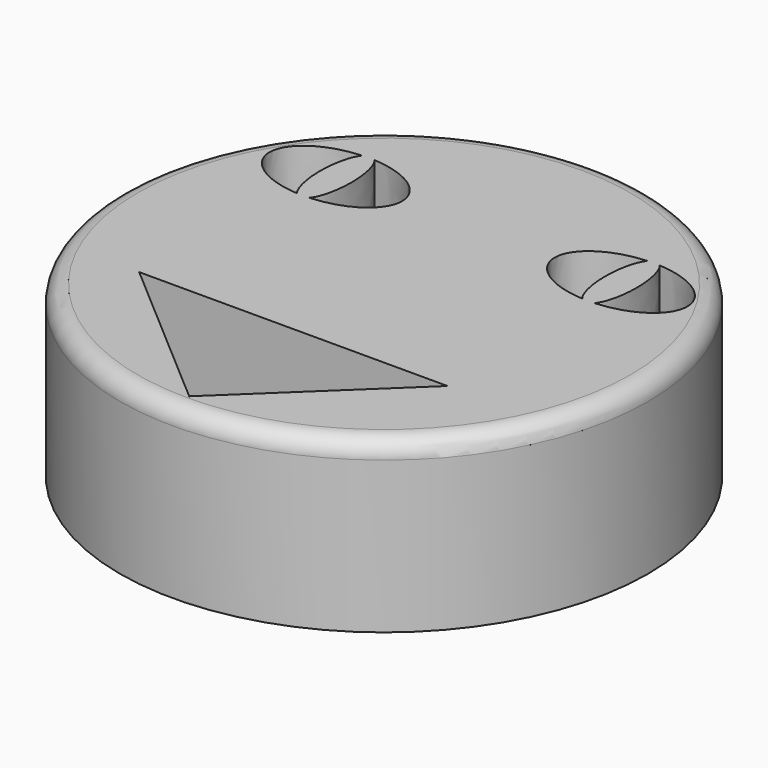
from build123d import *

# Parameters (mm, degrees)
F0_R     = 75.6558411923
F1_DEPTH = 48.514
F2_R     = 5.08


with BuildPart() as f1:
    # F0 (on Top) → F1 (new body)
    with BuildSketch(Plane.XY):
        Circle(F0_R)
        Polygon((0, -69.7530433536), (-46.3102683425, -29.7708865255), (41.9956482947, -29.7708865255), align=None, mode=Mode.SUBTRACT)
        with BuildLine():
            add(Edge.make_bspline(
                [(-21.8607485294, 33.7978675961), (-21.8607485294, 44.4959185344), (-39.0945518587, 45.4823768148)],
                knots=[0, 0, 0, 1.4784559967, 1.4784559967, 1.4784559967], degree=2, weights=[1, 0.73898889, 1]))
            add(Edge.make_bspline(
                [(-39.0945518587, 22.1133583775), (-21.8607485294, 23.0998166579), (-21.8607485294, 33.7978675961)],
                knots=[4.8047293104, 4.8047293104, 4.8047293104, 6.2831853072, 6.2831853072, 6.2831853072], degree=2, weights=[1, 0.73898889, 1]))
            add(Edge.make_bspline(
                [(-40.8450812101, 21.1076120934), (-39.9337015522, 21.1076120934), (-39.0945518587, 22.1133583775)],
                knots=[0, 0, 0, 0.4008066518, 0.4008066518, 0.4008066518], degree=2, weights=[1, 0.9799863696, 1]))
            add(Edge.make_bspline(
                [(-42.5956105616, 22.1133583775), (-41.7564608681, 21.1076120934), (-40.8450812101, 21.1076120934)],
                knots=[5.8823786554, 5.8823786554, 5.8823786554, 6.2831853072, 6.2831853072, 6.2831853072], degree=2, weights=[1, 0.9799863696, 1]))
            add(Edge.make_bspline(
                [(-42.5956105616, 45.4823768148), (-59.8294138908, 44.4959185344), (-59.8294138908, 33.7978675961), (-59.8294138908, 23.0998166579), (-42.5956105616, 22.1133583775)],
                knots=[1.6631366568, 1.6631366568, 1.6631366568, 3.1415926536, 3.1415926536, 4.6200486503, 4.6200486503, 4.6200486503], degree=2, weights=[1, 0.73898889, 1, 0.73898889, 1]))
            add(Edge.make_bspline(
                [(-39.0945518587, 45.4823768148), (-40.8450812101, 47.5804391797), (-42.5956105616, 45.4823768148)],
                knots=[2.7407860018, 2.7407860018, 2.7407860018, 3.5423993054, 3.5423993054, 3.5423993054], degree=2, weights=[1, 0.9207465694, 1]))
        make_face(mode=Mode.SUBTRACT)
        with BuildLine():
            add(Edge.make_bspline(
                [(21.8607485294, 33.7978675961), (21.8607485294, 23.0998166579), (39.0945518587, 22.1133583775)],
                knots=[0, 0, 0, 1.4784559967, 1.4784559967, 1.4784559967], degree=2, weights=[1, 0.73898889, 1]))
            add(Edge.make_bspline(
                [(39.0945518587, 45.4823768148), (21.8607485294, 44.4959185344), (21.8607485294, 33.7978675961)],
                knots=[4.8047293104, 4.8047293104, 4.8047293104, 6.2831853072, 6.2831853072, 6.2831853072], degree=2, weights=[1, 0.73898889, 1]))
            add(Edge.make_bspline(
                [(42.5956105616, 45.4823768148), (40.8450812101, 47.5804391797), (39.0945518587, 45.4823768148)],
                knots=[2.7407860018, 2.7407860018, 2.7407860018, 3.5423993054, 3.5423993054, 3.5423993054], degree=2, weights=[1, 0.9207465694, 1]))
            add(Edge.make_bspline(
                [(42.5956105616, 22.1133583775), (59.8294138908, 23.0998166579), (59.8294138908, 33.7978675961), (59.8294138908, 44.4959185344), (42.5956105616, 45.4823768148)],
                knots=[1.6631366568, 1.6631366568, 1.6631366568, 3.1415926536, 3.1415926536, 4.6200486503, 4.6200486503, 4.6200486503], degree=2, weights=[1, 0.73898889, 1, 0.73898889, 1]))
            add(Edge.make_bspline(
                [(40.8450812101, 21.1076120934), (41.7564608681, 21.1076120934), (42.5956105616, 22.1133583775)],
                knots=[0, 0, 0, 0.4008066518, 0.4008066518, 0.4008066518], degree=2, weights=[1, 0.9799863696, 1]))
            add(Edge.make_bspline(
                [(39.0945518587, 22.1133583775), (39.9337015522, 21.1076120934), (40.8450812101, 21.1076120934)],
                knots=[5.8823786554, 5.8823786554, 5.8823786554, 6.2831853072, 6.2831853072, 6.2831853072], degree=2, weights=[1, 0.9799863696, 1]))
        make_face(mode=Mode.SUBTRACT)
        with BuildLine():
            add(Edge.make_bspline(
                [(-39.0945518587, 22.1133583775), (-29.3455202344, 33.7978675961), (-39.0945518587, 45.4823768148)],
                knots=[0.4008066518, 0.4008066518, 0.4008066518, 2.7407860018, 2.7407860018, 2.7407860018], degree=2, weights=[1, 0.390161191, 1]))
            add(Edge.make_bspline(
                [(-39.0945518587, 45.4823768148), (-40.8450812101, 45.5825766454), (-42.5956105616, 45.4823768148)],
                knots=[1.4784559967, 1.4784559967, 1.4784559967, 1.6631366568, 1.6631366568, 1.6631366568], degree=2, weights=[1, 0.9957396602, 1]))
            add(Edge.make_bspline(
                [(-42.5956105616, 45.4823768148), (-52.3446421858, 33.7978675961), (-42.5956105616, 22.1133583775)],
                knots=[3.5423993054, 3.5423993054, 3.5423993054, 5.8823786554, 5.8823786554, 5.8823786554], degree=2, weights=[1, 0.390161191, 1]))
            add(Edge.make_bspline(
                [(-42.5956105616, 22.1133583775), (-40.8450812101, 22.0131585469), (-39.0945518587, 22.1133583775)],
                knots=[4.6200486503, 4.6200486503, 4.6200486503, 4.8047293104, 4.8047293104, 4.8047293104], degree=2, weights=[1, 0.9957396602, 1]))
        make_face()
        with BuildLine():
            add(Edge.make_bspline(
                [(-39.0945518587, 45.4823768148), (-40.8450812101, 45.5825766454), (-42.5956105616, 45.4823768148)],
                knots=[1.4784559967, 1.4784559967, 1.4784559967, 1.6631366568, 1.6631366568, 1.6631366568], degree=2, weights=[1, 0.9957396602, 1]))
            add(Edge.make_bspline(
                [(-39.0945518587, 45.4823768148), (-40.8450812101, 47.5804391797), (-42.5956105616, 45.4823768148)],
                knots=[2.7407860018, 2.7407860018, 2.7407860018, 3.5423993054, 3.5423993054, 3.5423993054], degree=2, weights=[1, 0.9207465694, 1]))
        make_face()
        with BuildLine():
            add(Edge.make_bspline(
                [(-40.8450812101, 21.1076120934), (-39.9337015522, 21.1076120934), (-39.0945518587, 22.1133583775)],
                knots=[0, 0, 0, 0.4008066518, 0.4008066518, 0.4008066518], degree=2, weights=[1, 0.9799863696, 1]))
            add(Edge.make_bspline(
                [(-42.5956105616, 22.1133583775), (-40.8450812101, 22.0131585469), (-39.0945518587, 22.1133583775)],
                knots=[4.6200486503, 4.6200486503, 4.6200486503, 4.8047293104, 4.8047293104, 4.8047293104], degree=2, weights=[1, 0.9957396602, 1]))
            add(Edge.make_bspline(
                [(-42.5956105616, 22.1133583775), (-41.7564608681, 21.1076120934), (-40.8450812101, 21.1076120934)],
                knots=[5.8823786554, 5.8823786554, 5.8823786554, 6.2831853072, 6.2831853072, 6.2831853072], degree=2, weights=[1, 0.9799863696, 1]))
        make_face()
        with BuildLine():
            add(Edge.make_bspline(
                [(39.0945518587, 45.4823768148), (29.3455202344, 33.7978675961), (39.0945518587, 22.1133583775)],
                knots=[3.5423993054, 3.5423993054, 3.5423993054, 5.8823786554, 5.8823786554, 5.8823786554], degree=2, weights=[1, 0.390161191, 1]))
            add(Edge.make_bspline(
                [(39.0945518587, 22.1133583775), (40.8450812101, 22.0131585469), (42.5956105616, 22.1133583775)],
                knots=[1.4784559967, 1.4784559967, 1.4784559967, 1.6631366568, 1.6631366568, 1.6631366568], degree=2, weights=[1, 0.9957396602, 1]))
            add(Edge.make_bspline(
                [(42.5956105616, 22.1133583775), (52.3446421858, 33.7978675961), (42.5956105616, 45.4823768148)],
                knots=[0.4008066518, 0.4008066518, 0.4008066518, 2.7407860018, 2.7407860018, 2.7407860018], degree=2, weights=[1, 0.390161191, 1]))
            add(Edge.make_bspline(
                [(42.5956105616, 45.4823768148), (40.8450812101, 45.5825766454), (39.0945518587, 45.4823768148)],
                knots=[4.6200486503, 4.6200486503, 4.6200486503, 4.8047293104, 4.8047293104, 4.8047293104], degree=2, weights=[1, 0.9957396602, 1]))
        make_face()
        with BuildLine():
            add(Edge.make_bspline(
                [(39.0945518587, 22.1133583775), (40.8450812101, 22.0131585469), (42.5956105616, 22.1133583775)],
                knots=[1.4784559967, 1.4784559967, 1.4784559967, 1.6631366568, 1.6631366568, 1.6631366568], degree=2, weights=[1, 0.9957396602, 1]))
            add(Edge.make_bspline(
                [(39.0945518587, 22.1133583775), (39.9337015522, 21.1076120934), (40.8450812101, 21.1076120934)],
                knots=[5.8823786554, 5.8823786554, 5.8823786554, 6.2831853072, 6.2831853072, 6.2831853072], degree=2, weights=[1, 0.9799863696, 1]))
            add(Edge.make_bspline(
                [(40.8450812101, 21.1076120934), (41.7564608681, 21.1076120934), (42.5956105616, 22.1133583775)],
                knots=[0, 0, 0, 0.4008066518, 0.4008066518, 0.4008066518], degree=2, weights=[1, 0.9799863696, 1]))
        make_face()
        with BuildLine():
            add(Edge.make_bspline(
                [(42.5956105616, 45.4823768148), (40.8450812101, 47.5804391797), (39.0945518587, 45.4823768148)],
                knots=[2.7407860018, 2.7407860018, 2.7407860018, 3.5423993054, 3.5423993054, 3.5423993054], degree=2, weights=[1, 0.9207465694, 1]))
            add(Edge.make_bspline(
                [(42.5956105616, 45.4823768148), (40.8450812101, 45.5825766454), (39.0945518587, 45.4823768148)],
                knots=[4.6200486503, 4.6200486503, 4.6200486503, 4.8047293104, 4.8047293104, 4.8047293104], degree=2, weights=[1, 0.9957396602, 1]))
        make_face()
    extrude(amount=F1_DEPTH)

    # F2
    f2_edges = [f1.edges().sort_by_distance(p)[0] for p in [
        (-75.655841, 0, 48.514),
    ]]
    fillet(f2_edges, radius=F2_R)


solid = f1.part
